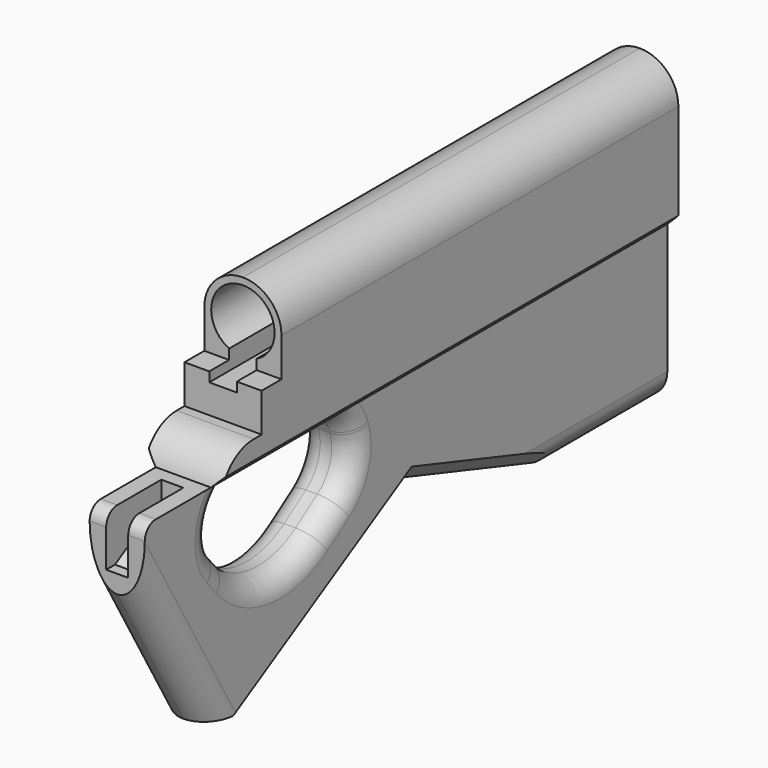
from build123d import *

# Parameters (mm, degrees)
F2_DEPTH      = 12.7
F3_DEPTH      = 5.08
F4_DEPTH      = 17.78
F5_SIZE       = 6.35
F6_F1_R       = 12.7
F6_F2_R       = 12.7
F6_F3_R       = 12.6999
F6_F4_R       = 12.6999
F7_R          = 17.77999
F8_DEPTH      = 279.4
F9_R          = 6.35
F10_SIZE      = 5.07999
F12_DEPTH     = 38.1
F13_T1_DEPTH  = 8.2086799032
F13_T3_DEPTH  = 15.1743095817
F13_T5_DEPTH  = 1.2682069324
F13_T10_ANGLE = 206.4656880666
F13_T15_ANGLE = 206.4656880666
F13_T18_ANGLE = 84.3612988267
F13_T20_ANGLE = 84.3612988267
F13_T22_ANGLE = 73.9106389354
F13_T24_ANGLE = 73.9106389354
F13_T28_ANGLE = 148.1491883443
F13_T33_ANGLE = 148.1491883443


# Not quite as in the source:
# - a fillet or chamfer that OpenCascade refuses, or shapes differently, is made with other operations: its cross-section is extruded or revolved along the edge and cut away or added
# - a fillet or chamfer is up to 0.001 mm smaller than in the source, because OpenCascade refuses the exact size


with BuildPart() as f2:
    # F1 (on Right) → F2 (new body, symmetric)
    with BuildSketch(Plane.YZ):
        Polygon((31.75, 0), (0, 0), (0, -23.622), (5.08, -23.622), (31.75, -8.255), align=None)
        Polygon((38.1, 0), (31.75, 0), (31.75, -8.255), (5.08, -23.622), (0, -23.622), (0, -31.9232071557), (38.1, -97.914342924), (63.5, -97.914342924), (154.4352262806, -45.4128655521), (237.49, -72.517), (300.99, -72.517), (300.99, 0), align=None)
    extrude(amount=F2_DEPTH, both=True)

    # F1 (on Right) → F3 (cut, symmetric)
    with BuildSketch(Plane.YZ):
        Polygon((31.75, 0), (0, 0), (0, -23.622), (5.08, -23.622), (31.75, -8.255), align=None)
    extrude(amount=F3_DEPTH, both=True, mode=Mode.SUBTRACT)

    # F1 (on Right) → F4 (join, symmetric)
    with BuildSketch(Plane.YZ):
        with BuildLine():
            ThreePointArc((56.4245641422, 13.843), (44.9417694039, 9.9932606886), (38.1, 0))
            Line((38.1, 0), (300.99, 0))
            Line((300.99, 0), (300.99, 67.183))
            Line((300.99, 67.183), (72.39, 67.183))
            Line((72.39, 67.183), (72.39, 49.403))
            Line((72.39, 49.403), (72.39, 31.623))
            Line((72.39, 31.623), (60.96, 31.623))
            Line((60.96, 31.623), (60.96, 13.843))
            Line((60.96, 13.843), (56.4245641422, 13.843))
        make_face()
    extrude(amount=F4_DEPTH, both=True)

    # F5
    f5_edges = [f2.edges().sort_by_distance(p)[0] for p in [
        (-12.7, 108.967613, -71.663604),
        (-12.7, 195.962613, -58.964933),
        (12.7, 108.967613, -71.663604),
        (12.7, 195.962613, -58.964933),
    ]]
    chamfer(f5_edges, length=F5_SIZE)

    # F6: fillet of radius 12.7 on 4 edges, made by hand

    # F6_f1
    f6_f1_edges = [f2.edges().sort_by_distance(p)[0] for p in [
        (12.7, 19.05, -64.9187750398),
    ]]
    fillet(f6_f1_edges, radius=F6_F1_R)

    # F6_f2
    f6_f2_edges = [f2.edges().sort_by_distance(p)[0] for p in [
        (12.7, 279.4740638835, -72.517),
    ]]
    fillet(f6_f2_edges, radius=F6_F2_R)

    # F6_f3 (radius 12.7 in the source; OpenCascade refuses exactly that, so slightly less here)
    f6_f3_edges = [f2.edges().sort_by_distance(p)[0] for p in [
        (-12.7, 19.05, -64.9187750398),
    ]]
    fillet(f6_f3_edges, radius=F6_F3_R)

    # F6_f4 (radius 12.7 in the source; OpenCascade refuses exactly that, so slightly less here)
    f6_f4_edges = [f2.edges().sort_by_distance(p)[0] for p in [
        (-12.7, 279.4740638835, -72.517),
    ]]
    fillet(f6_f4_edges, radius=F6_F4_R)

    # F7 (radius 17.78 in the source; OpenCascade refuses exactly that, so slightly less here)
    f7_edges = [f2.edges().sort_by_distance(p)[0] for p in [
        (17.78, 186.69, 67.183),
        (-17.78, 186.69, 67.183),
    ]]
    fillet(f7_edges, radius=F7_R)

    # F0 (on Front) → F8 (cut)
    with BuildSketch(Plane.XZ):
        with BuildLine():
            Line((6.35, 27.178), (6.35, 36.2506798625))
            ThreePointArc((6.35, 36.2506798625), (0, 64.008), (-6.35, 36.2506798625))
            Line((-6.35, 36.2506798625), (-6.35, 27.178))
            Line((-6.35, 27.178), (0, 27.178))
            Line((0, 27.178), (6.35, 27.178))
        make_face()
    extrude(amount=-F8_DEPTH, mode=Mode.SUBTRACT)

    # F9
    f9_edges = [f2.edges().sort_by_distance(p)[0] for p in [
        (8.89, 0, 0),
        (-8.89, 0, 0),
    ]]
    fillet(f9_edges, radius=F9_R)

    # F10 (size 5.08 in the source; OpenCascade refuses exactly that, so slightly less here)
    f10_edges = [f2.edges().sort_by_distance(p)[0] for p in [
        (17.78, 169.545, 0),
        (-17.78, 169.545, 0),
    ]]
    chamfer(f10_edges, length=F10_SIZE)

    # F11 (on Right) → F12 (cut, symmetric)
    with BuildSketch(Plane.YZ):
        with BuildLine():
            Line((100.8271926314, 0), (58.0769085959, 0))
            ThreePointArc((58.0769085959, 0), (40.8117452528, -10.9991221138), (43.4837619545, -31.2951039645))
            Line((43.4837619545, -31.2951039645), (48.7601996881, -37.5833175897))
            ThreePointArc((48.7601996881, -37.5833175897), (72.7629814409, -50.8388539005), (99.4504964842, -44.5444662753))
            Line((99.4504964842, -44.5444662753), (111.9768120232, -35.9799411689))
            ThreePointArc((111.9768120232, -35.9799411689), (119.2709367935, -26.3567064191), (119.3142930835, -14.2815656974))
            Line((119.3142930835, -14.2815656974), (118.9166754484, -13.0773028359))
            ThreePointArc((118.9166754484, -13.0773028359), (111.9878964404, -3.6116972925), (100.8271926314, 0))
        make_face()
    extrude(amount=F12_DEPTH, both=True, mode=Mode.SUBTRACT)

    # F13: fillet of radius 10.16 on 12 edges, made by hand

    # F13_s2 → F13_t1 (cut)
    with BuildSketch(Plane(origin=(0, 33.3762734743, -39.7762938204), x_dir=(1, 0, 0), z_dir=(0, 0.6427876097, -0.7660444431))):
        with BuildLine():
            ThreePointArc((2.5390343146, -13.1947891389), (9.7242048969, -10.2185940357), (12.7004, -3.0334234534))
            Line((12.7004, -3.0334234534), (13.7165365685, -3.0334234534))
            ThreePointArc((13.7165365685, -3.0334234534), (13.7161365685, -8.1139062962), (13.7161365685, -13.1943891389))
            Line((13.7161365685, -13.1943891389), (12.7, -14.2105257074))
            ThreePointArc((12.7, -14.2105257074), (7.6195171573, -14.2105257074), (2.5390343146, -14.2109257074))
            Line((2.5390343146, -14.2109257074), (2.5390343146, -13.1947891389))
        make_face()
        with BuildLine():
            ThreePointArc((-2.5390343146, -13.1947891389), (-9.7242048969, -10.2185940357), (-12.7004, -3.0334234534))
            Line((-12.7004, -3.0334234534), (-13.7165365685, -3.0334234534))
            ThreePointArc((-13.7165365685, -3.0334234534), (-13.7161365685, -8.1139062962), (-13.7161365685, -13.1943891389))
            Line((-13.7161365685, -13.1943891389), (-12.7, -14.2105257074))
            ThreePointArc((-12.7, -14.2105257074), (-7.6195171573, -14.2105257074), (-2.5390343146, -14.2109257074))
            Line((-2.5390343146, -14.2109257074), (-2.5390343146, -13.1947891389))
        make_face()
    extrude(amount=F13_T1_DEPTH, mode=Mode.SUBTRACT)

    # F13_s4 → F13_t3 (cut)
    with BuildSketch(Plane(origin=(0, 47.0156987889, 32.1456961085), x_dir=(1, 0, 0), z_dir=(0, 0.8254949243, 0.564409541))):
        with BuildLine():
            ThreePointArc((2.5390343146, 92.9016398904), (9.7242048969, 95.8778349935), (12.7004, 103.0630055758))
            Line((12.7004, 103.0630055758), (13.7165365685, 103.0630055758))
            ThreePointArc((13.7165365685, 103.0630055758), (13.7161365685, 97.9825227331), (13.7161365685, 92.9020398904))
            Line((13.7161365685, 92.9020398904), (12.7, 91.8859033218))
            ThreePointArc((12.7, 91.8859033218), (7.6195171573, 91.8859033218), (2.5390343146, 91.8855033218))
            Line((2.5390343146, 91.8855033218), (2.5390343146, 92.9016398904))
        make_face()
        with BuildLine():
            ThreePointArc((-2.5390343146, 92.9016398904), (-9.7242048969, 95.8778349935), (-12.7004, 103.0630055758))
            Line((-12.7004, 103.0630055758), (-13.7165365685, 103.0630055758))
            ThreePointArc((-13.7165365685, 103.0630055758), (-13.7161365685, 97.9825227331), (-13.7161365685, 92.9020398904))
            Line((-13.7161365685, 92.9020398904), (-12.7, 91.8859033218))
            ThreePointArc((-12.7, 91.8859033218), (-7.6195171573, 91.8859033218), (-2.5390343146, 91.8855033218))
            Line((-2.5390343146, 91.8855033218), (-2.5390343146, 92.9016398904))
        make_face()
    extrude(amount=F13_T3_DEPTH, mode=Mode.SUBTRACT)

    # F13_s6 → F13_t5 (cut)
    with BuildSketch(Plane(origin=(0, 15.9804225983, -48.3998388094), x_dir=(1, 0, 0), z_dir=(0, -0.3135274102, 0.9495791505))):
        with BuildLine():
            ThreePointArc((2.5390343146, 108.8203027619), (9.7242048969, 111.796497865), (12.7004, 118.9816684473))
            Line((12.7004, 118.9816684473), (13.7165365685, 118.9816684473))
            ThreePointArc((13.7165365685, 118.9816684473), (13.7161365685, 113.9011856046), (13.7161365685, 108.8207027619))
            Line((13.7161365685, 108.8207027619), (12.7, 107.8045661934))
            ThreePointArc((12.7, 107.8045661934), (7.6195171573, 107.8045661934), (2.5390343146, 107.8041661934))
            Line((2.5390343146, 107.8041661934), (2.5390343146, 108.8203027619))
        make_face()
        with BuildLine():
            ThreePointArc((-2.5390343146, 108.8203027619), (-9.7242048969, 111.796497865), (-12.7004, 118.9816684473))
            Line((-12.7004, 118.9816684473), (-13.7165365685, 118.9816684473))
            ThreePointArc((-13.7165365685, 118.9816684473), (-13.7161365685, 113.9011856046), (-13.7161365685, 108.8207027619))
            Line((-13.7161365685, 108.8207027619), (-12.7, 107.8045661934))
            ThreePointArc((-12.7, 107.8045661934), (-7.6195171573, 107.8045661934), (-2.5390343146, 107.8041661934))
            Line((-2.5390343146, 107.8041661934), (-2.5390343146, 108.8203027619))
        make_face()
    extrude(amount=F13_T5_DEPTH, mode=Mode.SUBTRACT)


with BuildPart() as f13_tool8:
    # F13_s9 → F13_t10 (revolve)
    with BuildSketch(Plane(origin=(0, 7.5152314778, -31.2208137079), x_dir=(1, 0, 0), z_dir=(0, 0.2340276317, -0.9722299458))):
        with BuildLine():
            ThreePointArc((2.5390343146, -71.0554833143), (9.7242048969, -74.0316784175), (12.7004, -81.2168489997))
            Line((12.7004, -81.2168489997), (13.7165365685, -81.2168489997))
            ThreePointArc((13.7165365685, -81.2168489997), (13.7161365685, -76.136366157), (13.7161365685, -71.0558833143))
            Line((13.7161365685, -71.0558833143), (12.7, -70.0397467458))
            ThreePointArc((12.7, -70.0397467458), (7.6195171573, -70.0397467458), (2.5390343146, -70.0393467458))
            Line((2.5390343146, -70.0393467458), (2.5390343146, -71.0554833143))
        make_face()
    revolve(axis=Axis((12.7, 58.0769085959, -19.05), (1, 0, 0)), revolution_arc=F13_T10_ANGLE)

    split(bisect_by=Plane.XY, keep=Keep.BOTTOM)


with BuildPart() as f2_1:
    add(f2.part)

    # F13_t7: cut F13_tool8
    add(f13_tool8.part, mode=Mode.SUBTRACT)


with BuildPart() as f13_tool13:
    # F13_s14 → F13_t15 (revolve)
    with BuildSketch(Plane(origin=(0, 7.5152314778, -31.2208137079), x_dir=(1, 0, 0), z_dir=(0, 0.2340276317, -0.9722299458))):
        with BuildLine():
            ThreePointArc((-2.5390343146, -71.0554833143), (-9.7242048969, -74.0316784175), (-12.7004, -81.2168489997))
            Line((-12.7004, -81.2168489997), (-13.7165365685, -81.2168489997))
            ThreePointArc((-13.7165365685, -81.2168489997), (-13.7161365685, -76.136366157), (-13.7161365685, -71.0558833143))
            Line((-13.7161365685, -71.0558833143), (-12.7, -70.0397467458))
            ThreePointArc((-12.7, -70.0397467458), (-7.6195171573, -70.0397467458), (-2.5390343146, -70.0393467458))
            Line((-2.5390343146, -70.0393467458), (-2.5390343146, -71.0554833143))
        make_face()
    revolve(axis=Axis((-12.7, 58.0769085959, -19.05), (1, 0, 0)), revolution_arc=F13_T15_ANGLE)

    split(bisect_by=Plane.XY, keep=Keep.BOTTOM)


with BuildPart() as f2_2:
    add(f2_1.part)

    # F13_t12: cut F13_tool13
    add(f13_tool13.part, mode=Mode.SUBTRACT)

    # F13_s17 → F13_t18 (revolve, cut)
    with BuildSketch(Plane(origin=(0, 38.6527112079, -46.0645074456), x_dir=(1, 0, 0), z_dir=(0, -0.6427876097, 0.7660444431))):
        with BuildLine():
            ThreePointArc((2.5390343146, 13.1947891389), (9.7242048969, 10.2185940357), (12.7004, 3.0334234534))
            Line((12.7004, 3.0334234534), (13.7165365685, 3.0334234534))
            ThreePointArc((13.7165365685, 3.0334234534), (13.7161365685, 8.1139062962), (13.7161365685, 13.1943891389))
            Line((13.7161365685, 13.1943891389), (12.7, 14.2105257074))
            ThreePointArc((12.7, 14.2105257074), (7.6195171573, 14.2105257074), (2.5390343146, 14.2109257074))
            Line((2.5390343146, 14.2109257074), (2.5390343146, 13.1947891389))
        make_face()
    revolve(axis=Axis((12.7, 77.9464929709, -13.0931096607), (1, 0, 0)), revolution_arc=F13_T18_ANGLE, mode=Mode.SUBTRACT)

    # F13_s19 → F13_t20 (revolve, cut)
    with BuildSketch(Plane(origin=(0, 38.6527112079, -46.0645074456), x_dir=(1, 0, 0), z_dir=(0, -0.6427876097, 0.7660444431))):
        with BuildLine():
            ThreePointArc((-2.5390343146, 13.1947891389), (-9.7242048969, 10.2185940357), (-12.7004, 3.0334234534))
            Line((-12.7004, 3.0334234534), (-13.7165365685, 3.0334234534))
            ThreePointArc((-13.7165365685, 3.0334234534), (-13.7161365685, 8.1139062962), (-13.7161365685, 13.1943891389))
            Line((-13.7161365685, 13.1943891389), (-12.7, 14.2105257074))
            ThreePointArc((-12.7, 14.2105257074), (-7.6195171573, 14.2105257074), (-2.5390343146, 14.2109257074))
            Line((-2.5390343146, 14.2109257074), (-2.5390343146, 13.1947891389))
        make_face()
    revolve(axis=Axis((-12.7, 77.9464929709, -13.0931096607), (1, 0, 0)), revolution_arc=F13_T20_ANGLE, mode=Mode.SUBTRACT)

    # F13_s21 → F13_t22 (revolve, cut)
    with BuildSketch(Plane(origin=(0, 59.5420143279, 40.7102212149), x_dir=(1, 0, 0), z_dir=(0, -0.8254949243, -0.564409541))):
        with BuildLine():
            ThreePointArc((2.5390343146, -92.9016398904), (9.7242048969, -95.8778349935), (12.7004, -103.0630055758))
            Line((12.7004, -103.0630055758), (13.7165365685, -103.0630055758))
            ThreePointArc((13.7165365685, -103.0630055758), (13.7161365685, -97.9825227331), (13.7161365685, -92.9020398904))
            Line((13.7161365685, -92.9020398904), (12.7, -91.8859033218))
            ThreePointArc((12.7, -91.8859033218), (7.6195171573, -91.8859033218), (2.5390343146, -91.8855033218))
            Line((2.5390343146, -91.8855033218), (2.5390343146, -92.9016398904))
        make_face()
    revolve(axis=Axis((12.7, 101.2248102665, -20.2542628615), (1, 0, 0)), revolution_arc=F13_T22_ANGLE, mode=Mode.SUBTRACT)

    # F13_s23 → F13_t24 (revolve, cut)
    with BuildSketch(Plane(origin=(0, 59.5420143279, 40.7102212149), x_dir=(1, 0, 0), z_dir=(0, -0.8254949243, -0.564409541))):
        with BuildLine():
            ThreePointArc((-2.5390343146, -92.9016398904), (-9.7242048969, -95.8778349935), (-12.7004, -103.0630055758))
            Line((-12.7004, -103.0630055758), (-13.7165365685, -103.0630055758))
            ThreePointArc((-13.7165365685, -103.0630055758), (-13.7161365685, -97.9825227331), (-13.7161365685, -92.9020398904))
            Line((-13.7161365685, -92.9020398904), (-12.7, -91.8859033218))
            ThreePointArc((-12.7, -91.8859033218), (-7.6195171573, -91.8859033218), (-2.5390343146, -91.8855033218))
            Line((-2.5390343146, -91.8855033218), (-2.5390343146, -92.9016398904))
        make_face()
    revolve(axis=Axis((-12.7, 101.2248102665, -20.2542628615), (1, 0, 0)), revolution_arc=F13_T24_ANGLE, mode=Mode.SUBTRACT)


with BuildPart() as f13_tool26:
    # F13_s27 → F13_t28 (revolve)
    with BuildSketch(Plane(origin=(0, 15.5828049632, -47.1955759479), x_dir=(1, 0, 0), z_dir=(0, 0.3135274102, -0.9495791505))):
        with BuildLine():
            ThreePointArc((-2.5390343146, -108.8203027619), (-9.7242048969, -111.796497865), (-12.7004, -118.9816684473))
            Line((-12.7004, -118.9816684473), (-13.7165365685, -118.9816684473))
            ThreePointArc((-13.7165365685, -118.9816684473), (-13.7161365685, -113.9011856046), (-13.7161365685, -108.8207027619))
            Line((-13.7161365685, -108.8207027619), (-12.7, -107.8045661934))
            ThreePointArc((-12.7, -107.8045661934), (-7.6195171573, -107.8045661934), (-2.5390343146, -107.8041661934))
            Line((-2.5390343146, -107.8041661934), (-2.5390343146, -108.8203027619))
        make_face()
    revolve(axis=Axis((-12.7, 100.8271926314, -19.05), (1, 0, 0)), revolution_arc=F13_T28_ANGLE)

    split(bisect_by=Plane.XY, keep=Keep.BOTTOM)


with BuildPart() as f2_3:
    add(f2_2.part)

    # F13_t25: cut F13_tool26
    add(f13_tool26.part, mode=Mode.SUBTRACT)


with BuildPart() as f13_tool31:
    # F13_s32 → F13_t33 (revolve)
    with BuildSketch(Plane(origin=(0, 15.5828049632, -47.1955759479), x_dir=(1, 0, 0), z_dir=(0, 0.3135274102, -0.9495791505))):
        with BuildLine():
            ThreePointArc((12.7004, -118.9816684473), (9.7242048969, -111.796497865), (2.5390343146, -108.8203027619))
            Line((2.5390343146, -108.8203027619), (2.5390343146, -107.8041661934))
            ThreePointArc((2.5390343146, -107.8041661934), (7.6195171573, -107.8045661934), (12.7, -107.8045661934))
            Line((12.7, -107.8045661934), (13.7161365685, -108.8207027619))
            ThreePointArc((13.7161365685, -108.8207027619), (13.7161365685, -113.9011856046), (13.7165365685, -118.9816684473))
            Line((13.7165365685, -118.9816684473), (12.7004, -118.9816684473))
        make_face()
    revolve(axis=Axis((12.7, 100.8271926314, -19.05), (1, 0, 0)), revolution_arc=F13_T33_ANGLE)

    split(bisect_by=Plane.XY, keep=Keep.BOTTOM)


with BuildPart() as f2_4:
    add(f2_3.part)

    # F13_t30: cut F13_tool31
    add(f13_tool31.part, mode=Mode.SUBTRACT)


solid = f2_4.part
